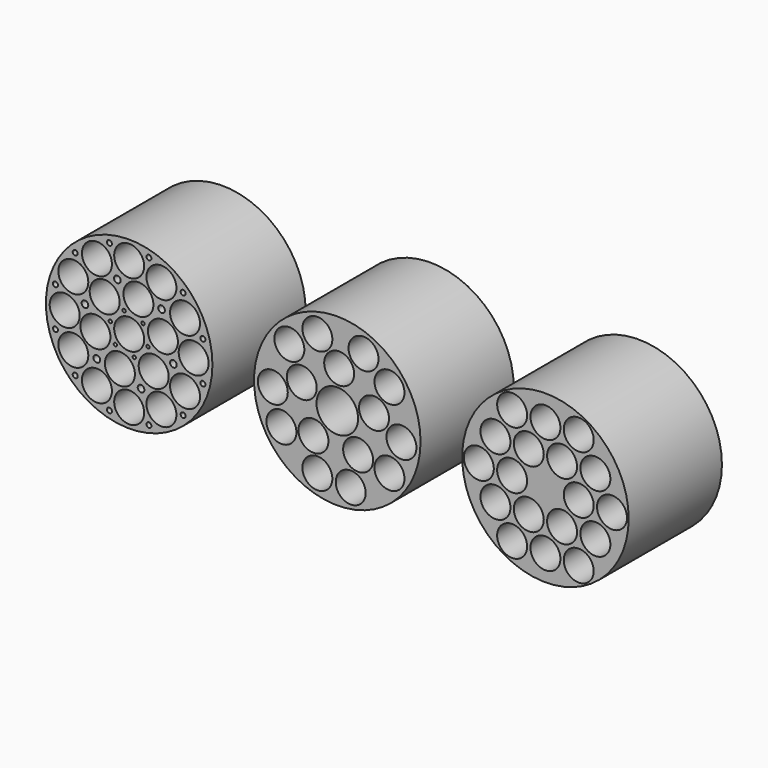
from build123d import *

# Parameters (mm, degrees)
F1_R      = 50
F1_R_2    = 9
F2_DEPTH  = 70
F0_R      = 50
F0_R_2    = 9
F4_DEPTH  = 70
F6_R      = 50
F6_R_2    = 9
F6_R_3    = 12.5
F7_DEPTH  = 70
F9_R      = 2
F9_R_2    = 1.5
F9_R_3    = 1
F10_DEPTH = 70.001


# Not quite as in the source:
# - the program builds the solid bodies; features that only make, move or delete a surface that nothing else refers to are left out


with BuildPart() as f2:
    # F1 (on Front) → F2 (new body)
    with BuildSketch(Plane.XZ):
        Circle(F1_R)
        with Locations((-20, -34.6410161514)):
            Circle(F1_R_2, mode=Mode.SUBTRACT)
        with Locations((-30, -17.3205080757)):
            Circle(F1_R_2, mode=Mode.SUBTRACT)
        with Locations((-10, -17.3205080757)):
            Circle(F1_R_2, mode=Mode.SUBTRACT)
        with Locations((0, -34.6410161514)):
            Circle(F1_R_2, mode=Mode.SUBTRACT)
        with Locations((20, -34.6410161514)):
            Circle(F1_R_2, mode=Mode.SUBTRACT)
        with Locations((10, -17.3205080757)):
            Circle(F1_R_2, mode=Mode.SUBTRACT)
        with Locations((30, -17.3205080757)):
            Circle(F1_R_2, mode=Mode.SUBTRACT)
        with Locations((-40, 0)):
            Circle(F1_R_2, mode=Mode.SUBTRACT)
        with Locations((-30, 17.3205080757)):
            Circle(F1_R_2, mode=Mode.SUBTRACT)
        with Locations((-20, 0)):
            Circle(F1_R_2, mode=Mode.SUBTRACT)
        with Locations((-10, 17.3205080757)):
            Circle(F1_R_2, mode=Mode.SUBTRACT)
        with Locations((-20, 34.6410161514)):
            Circle(F1_R_2, mode=Mode.SUBTRACT)
        with Locations((20, 0)):
            Circle(F1_R_2, mode=Mode.SUBTRACT)
        with Locations((10, 17.3205080757)):
            Circle(F1_R_2, mode=Mode.SUBTRACT)
        with Locations((40, 0)):
            Circle(F1_R_2, mode=Mode.SUBTRACT)
        with Locations((30, 17.3205080757)):
            Circle(F1_R_2, mode=Mode.SUBTRACT)
        with Locations((0, 34.6410161514)):
            Circle(F1_R_2, mode=Mode.SUBTRACT)
        with Locations((20, 34.6410161514)):
            Circle(F1_R_2, mode=Mode.SUBTRACT)
    extrude(amount=F2_DEPTH)


with BuildPart() as f2_1:
    # F3: moved
    add(f2.part.moved(Location((125, 0, 0))))


with BuildPart() as f4:
    # F0 (on Front) → F4 (new body)
    with BuildSketch(Plane.XZ):
        Circle(F0_R)
        with Locations((-19.3703155965, -33.5503707717)):
            Circle(F0_R_2, mode=Mode.SUBTRACT)
        with Locations((-33.5503707717, -19.3703155965)):
            Circle(F0_R_2, mode=Mode.SUBTRACT)
        with Locations((-5.5578491296, -20.2049845351)):
            Circle(F0_R_2, mode=Mode.SUBTRACT)
        with Locations((-20.2769544553, -5.2892537309)):
            Circle(F0_R_2, mode=Mode.SUBTRACT)
        with Locations((0, -38.7406311929)):
            Circle(F0_R_2, mode=Mode.SUBTRACT)
        with Locations((19.3703155965, -33.5503707717)):
            Circle(F0_R_2, mode=Mode.SUBTRACT)
        with Locations((14.7191053256, -14.9157308042)):
            Circle(F0_R_2, mode=Mode.SUBTRACT)
        with Locations((33.5503707717, -19.3703155965)):
            Circle(F0_R_2, mode=Mode.SUBTRACT)
        with Locations((-38.7406311929, 0)):
            Circle(F0_R_2, mode=Mode.SUBTRACT)
        with Locations((-33.5503707717, 19.3703155965)):
            Circle(F0_R_2, mode=Mode.SUBTRACT)
        with Locations((-14.7191053256, 14.9157308042)):
            Circle(F0_R_2, mode=Mode.SUBTRACT)
        with Locations((-19.3703155965, 33.5503707717)):
            Circle(F0_R_2, mode=Mode.SUBTRACT)
        Circle(F0_R_2, mode=Mode.SUBTRACT)
        with Locations((20.2769544553, 5.2892537309)):
            Circle(F0_R_2, mode=Mode.SUBTRACT)
        with Locations((5.5578491296, 20.2049845351)):
            Circle(F0_R_2, mode=Mode.SUBTRACT)
        with Locations((38.7406311929, 0)):
            Circle(F0_R_2, mode=Mode.SUBTRACT)
        with Locations((33.5503707717, 19.3703155965)):
            Circle(F0_R_2, mode=Mode.SUBTRACT)
        with Locations((19.3703155965, 33.5503707717)):
            Circle(F0_R_2, mode=Mode.SUBTRACT)
        with Locations((0, 38.7406311929)):
            Circle(F0_R_2, mode=Mode.SUBTRACT)
    extrude(amount=F4_DEPTH)


with BuildPart() as f4_1:
    # F5: moved
    add(f4.part.moved(Location((-125, 0, 0))))

    # F9 (on face) → F10 (cut, through all)
    with BuildSketch(Plane.XZ.offset(70)):
        with Locations((-151.5698701307, 7.1193752445)):
            Circle(F9_R)
        with Locations((-144.4504948862, -19.4504948862)):
            Circle(F9_R)
        with Locations((-117.8806247555, -26.5698701307)):
            Circle(F9_R)
        with Locations((-98.4301298693, -7.1193752445)):
            Circle(F9_R)
        with Locations((-105.5495051138, 19.4504948862)):
            Circle(F9_R)
        with Locations((-132.1193752445, 26.5698701307)):
            Circle(F9_R)
        with Locations((-169.2776831768, 11.8641694499)):
            Circle(F9_R_2)
        with Locations((-169.2776831768, -11.8641694499)):
            Circle(F9_R_2)
        with Locations((-157.4135137269, -32.4135137269)):
            Circle(F9_R_2)
        with Locations((-136.8641694499, -44.2776831768)):
            Circle(F9_R_2)
        with Locations((-113.1358305501, -44.2776831768)):
            Circle(F9_R_2)
        with Locations((-92.5864862731, -32.4135137269)):
            Circle(F9_R_2)
        with Locations((-80.7223168232, -11.8641694499)):
            Circle(F9_R_2)
        with Locations((-80.7223168232, 11.8641694499)):
            Circle(F9_R_2)
        with Locations((-92.5864862731, 32.4135137269)):
            Circle(F9_R_2)
        with Locations((-113.1358305501, 44.2776831768)):
            Circle(F9_R_2)
        with Locations((-136.8641694499, 44.2776831768)):
            Circle(F9_R_2)
        with Locations((-157.4135137269, 32.4135137269)):
            Circle(F9_R_2)
        with Locations((-136.3270046628, 3.0350617521)):
            Circle(F9_R_3)
        with Locations((-133.2919429108, -8.2919429108)):
            Circle(F9_R_3)
        with Locations((-121.9649382479, -11.3270046628)):
            Circle(F9_R_3)
        with Locations((-113.6729953372, -3.0350617521)):
            Circle(F9_R_3)
        with Locations((-116.7080570892, 8.2919429108)):
            Circle(F9_R_3)
        with Locations((-128.0350617521, 11.3270046628)):
            Circle(F9_R_3)
    extrude(amount=-F10_DEPTH, mode=Mode.SUBTRACT)


with BuildPart() as f7:
    # F6 (on Front) → F7 (new body)
    with BuildSketch(Plane.XZ):
        Circle(F6_R)
        with Locations((-11.9715134114, -36.8445297414)):
            Circle(F6_R_2, mode=Mode.SUBTRACT)
        with Locations((-33.5503707717, -19.3703155965)):
            Circle(F6_R_2, mode=Mode.SUBTRACT)
        with Locations((-14.3274884058, -17.8011459818)):
            Circle(F6_R_2, mode=Mode.SUBTRACT)
        with Locations((8.0546301347, -37.8940554523)):
            Circle(F6_R_2, mode=Mode.SUBTRACT)
        with Locations((12.5024584794, -19.1271078382)):
            Circle(F6_R_2, mode=Mode.SUBTRACT)
        with Locations((31.3418290079, -22.7711716797)):
            Circle(F6_R_2, mode=Mode.SUBTRACT)
        with Locations((38.5284059617, -4.0494986446)):
            Circle(F6_R_2, mode=Mode.SUBTRACT)
        with Locations((-38.7406311929, 0)):
            Circle(F6_R_2, mode=Mode.SUBTRACT)
        with Locations((-21.3573332876, 8.1253945827)):
            Circle(F6_R_2, mode=Mode.SUBTRACT)
        with Locations((-28.7898996067, 25.9225420408)):
            Circle(F6_R_2, mode=Mode.SUBTRACT)
        with Locations((-11.9715134114, 36.8445297414)):
            Circle(F6_R_2, mode=Mode.SUBTRACT)
        Circle(F6_R_3, mode=Mode.SUBTRACT)
        with Locations((22.054432689, 5.9799432313)):
            Circle(F6_R_2, mode=Mode.SUBTRACT)
        with Locations((1.127930525, 22.8229160059)):
            Circle(F6_R_2, mode=Mode.SUBTRACT)
        with Locations((31.3418290079, 22.7711716797)):
            Circle(F6_R_2, mode=Mode.SUBTRACT)
        with Locations((15.757234282, 35.3913276525)):
            Circle(F6_R_2, mode=Mode.SUBTRACT)
    extrude(amount=F7_DEPTH)


solid = Compound([f2_1.part, f4_1.part, f7.part])
